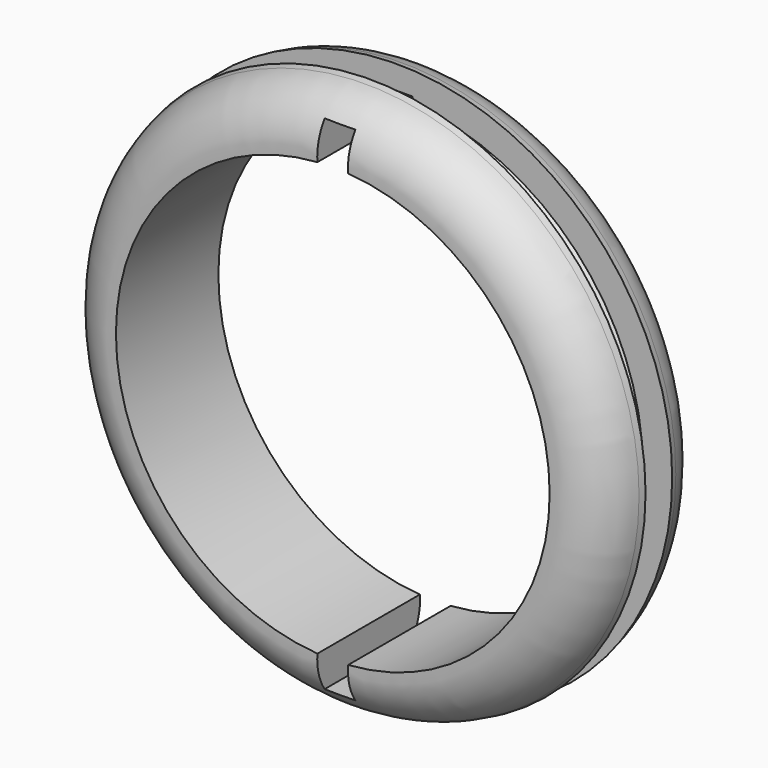
from build123d import *

# Parameters (mm, degrees)
F4_W          = 1.2
F4_H          = 19.620869044
F5_DEPTH      = 25
F5_DEPTH_BACK = 25


# Not quite as in the source:
# - a fillet or chamfer that OpenCascade refuses, or shapes differently, is made with other operations: its cross-section is extruded or revolved along the edge and cut away or added


with BuildPart() as f2:
    # F2: sweep along a path in F0
    with BuildLine(Plane.XZ) as f2_path:
        CenterArc((0, 0), 8.875, 0, 360)
    # F1 (on Right) → F2 (sweep)
    with BuildSketch(Plane.YZ):
        Polygon((-2.5, 8.4675319269), (0, 8.4675319269), (2.5, 8.4675319269), (2.7924242295, 10.246030055), (0.65, 10.7327634469), (0.65, 9.5877971399), (0.494154765, 9.4675319269), (0, 9.4675319269), (-0.494154765, 9.4675319269), (-0.65, 9.5877971399), (-0.65, 10.7327634469), (-2.7924242295, 10.246030055), align=None)
    sweep(path=f2_path.line)

    # F3: fillet of radius 2.0708896165 on 2 edges, made by hand

    # F3_s1 → F3_t2 (revolve, cut)
    with BuildSketch(Plane.XY):
        with BuildLine():
            ThreePointArc((10.6767355553, -0.8966145009), (9.8737027886, -2.1138201975), (8.4675319269, -2.5))
            Line((8.4675319269, -2.5), (10.246030055, -2.7924242295))
            Line((10.246030055, -2.7924242295), (10.6767355553, -0.8966145009))
        make_face()
    revolve(axis=Axis((0, -2.7924242295, 0), (0, -1, 0)), mode=Mode.SUBTRACT)

    # F3_s3 → F3_t4 (revolve, cut)
    with BuildSketch(Plane.XY):
        with BuildLine():
            ThreePointArc((8.4675319269, 2.5), (9.8737027886, 2.1138201975), (10.6767355553, 0.8966145009))
            Line((10.6767355553, 0.8966145009), (10.246030055, 2.7924242295))
            Line((10.246030055, 2.7924242295), (8.4675319269, 2.5))
        make_face()
    revolve(axis=Axis((0, 2.7924242295, 0), (0, -1, 0)), mode=Mode.SUBTRACT)

    # F4 (on Front) → F5 (cut, two sides)
    with BuildSketch(Plane.XZ) as f5_sk:
        Rectangle(F4_W, F4_H)
    extrude(amount=-F5_DEPTH, mode=Mode.SUBTRACT)
    extrude(f5_sk.sketch, amount=F5_DEPTH_BACK, mode=Mode.SUBTRACT)


solid = f2.part
